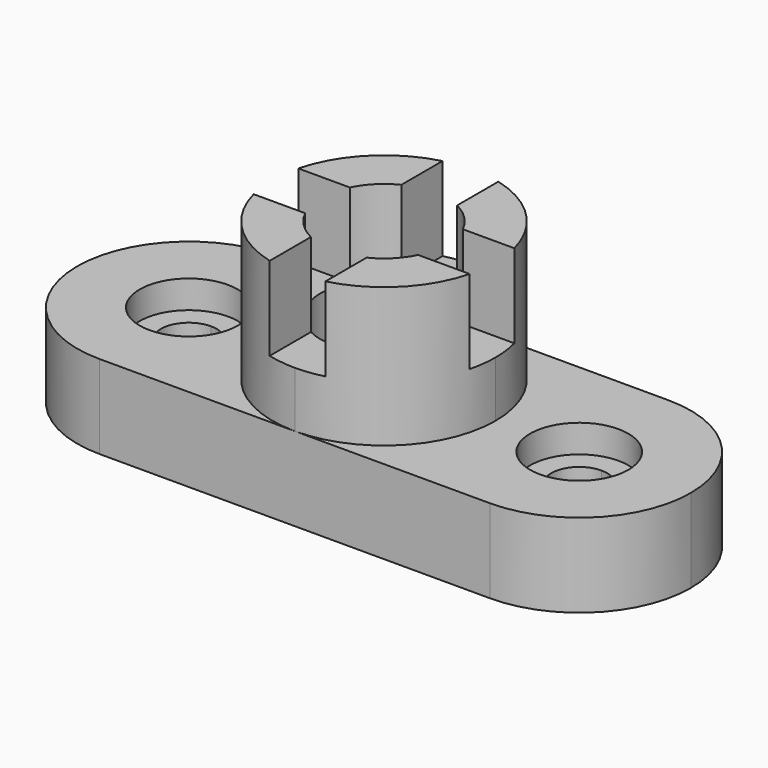
from build123d import *

# Parameters (mm, degrees)
F0_W      = 25.4
F0_H      = 31.75
F1_DEPTH  = 50.8
F2_R      = 14.351
F3_DEPTH  = 101.6
F4_W      = 12.7
F4_H      = 19.05
F5_DEPTH  = 254
F6_W      = 12.7
F6_H      = 19.05
F7_DEPTH  = 127
F9_DEPTH  = 6.35
F11_DEPTH = 6.35
F13_DEPTH = 50.8
F15_DEPTH = 558.8
F16_R     = 25.39999


# Not quite as in the source:
# - a fillet or chamfer is up to 0.001 mm smaller than in the source, because OpenCascade refuses the exact size


with BuildPart() as f1:
    # F0 (on Front) → F1 (new body)
    with BuildSketch(Plane.XZ):
        Polygon((0, 19.05), (0, 0), (139.7, 0), (139.7, 19.05), (95.25, 19.05), (69.85, 19.05), (44.45, 19.05), align=None)
        with Locations((57.15, 34.925)):
            Rectangle(F0_W, F0_H)
        with Locations((82.55, 34.925)):
            Rectangle(F0_W, F0_H)
    extrude(amount=F1_DEPTH)

    # F2 (on face) → F3 (cut)
    with BuildSketch(Plane.XY.offset(50.8)):
        with Locations((69.85, -25.4)):
            Circle(F2_R)
    extrude(amount=-F3_DEPTH, mode=Mode.SUBTRACT)

    # F4 (on face) → F5 (cut)
    with BuildSketch(Plane.XZ.offset(50.8)):
        with Locations((69.85, 41.275)):
            Rectangle(F4_W, F4_H)
    extrude(amount=-F5_DEPTH, mode=Mode.SUBTRACT)

    # F6 (on face) → F7 (cut)
    with BuildSketch(Plane.YZ.offset(95.25)):
        with Locations((-25.4, 41.275)):
            Rectangle(F6_W, F6_H)
    extrude(amount=-F7_DEPTH, mode=Mode.SUBTRACT)

    # F8 (on face) → F9 (cut)
    with BuildSketch(Plane.XY.offset(19.05)):
        with BuildLine():
            ThreePointArc((114.3, -36.576), (122.2026253865, -33.3026253865), (125.476, -25.4))
            ThreePointArc((125.476, -25.4), (106.3973746135, -17.4973746135), (114.3, -36.576))
        make_face()
    extrude(amount=-F9_DEPTH, mode=Mode.SUBTRACT)

    # F10 (on face) → F11 (cut)
    with BuildSketch(Plane.XY.offset(19.05)):
        with BuildLine():
            ThreePointArc((25.4, -36.576), (33.3026253865, -33.3026253865), (36.576, -25.4))
            ThreePointArc((36.576, -25.4), (17.4973746135, -17.4973746135), (25.4, -36.576))
        make_face()
    extrude(amount=-F11_DEPTH, mode=Mode.SUBTRACT)

    # F12 (on face) → F13 (cut)
    with BuildSketch(Plane(origin=(0, 0, 0), x_dir=(1, 0, 0), z_dir=(0, 0, -1))):
        with BuildLine():
            ThreePointArc((25.4, 19.05), (29.8901280605, 20.9098719395), (31.75, 25.4))
            ThreePointArc((31.75, 25.4), (20.9098719395, 29.8901280605), (25.4, 19.05))
        make_face()
    extrude(amount=-F13_DEPTH, mode=Mode.SUBTRACT)

    # F14 (on face) → F15 (cut)
    with BuildSketch(Plane(origin=(0, 0, 0), x_dir=(1, 0, 0), z_dir=(0, 0, -1))):
        with BuildLine():
            ThreePointArc((114.3, 19.05), (118.7901280605, 20.9098719395), (120.65, 25.4))
            ThreePointArc((120.65, 25.4), (109.8098719395, 29.8901280605), (114.3, 19.05))
        make_face()
    extrude(amount=-F15_DEPTH, mode=Mode.SUBTRACT)

    # F16 (radius 25.4 in the source; OpenCascade refuses exactly that, so slightly less here)
    f16_edges = [f1.edges().sort_by_distance(p)[0] for p in [
        (95.25, 0, 34.925),
        (95.25, -50.8, 34.925),
        (44.45, 0, 34.925),
        (44.45, -50.8, 34.925),
        (0, -50.8, 9.525),
        (0, 0, 9.525),
        (139.7, -50.8, 9.525),
        (139.7, 0, 9.525),
    ]]
    fillet(f16_edges, radius=F16_R)


solid = f1.part
